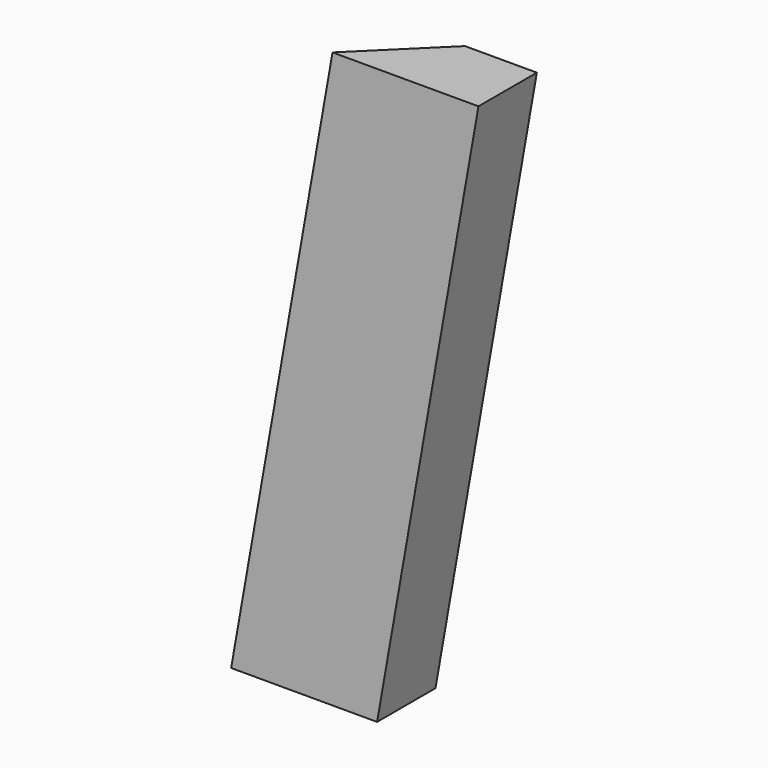
from build123d import *

# Parameters (mm, degrees)
F1_DEPTH = 20
F2_SIZE  = 19.99999


# Not quite as in the source:
# - a fillet or chamfer is up to 0.001 mm smaller than in the source, because OpenCascade refuses the exact size


with BuildPart() as f1:
    # F0 (on Front) → F1 (new body)
    with BuildSketch(Plane.XZ):
        Polygon((-27.7837084267, -157.569240482), (0, 0), (-40, 0), (-67.7837084267, -157.569240482), align=None)
    extrude(amount=F1_DEPTH)

    # F2 (size 20 in the source; OpenCascade refuses exactly that, so slightly less here)
    f2_edges = [f1.edges().sort_by_distance(p)[0] for p in [
        (-53.891854, 0, -78.78462),
    ]]
    chamfer(f2_edges, length=F2_SIZE)


solid = f1.part
